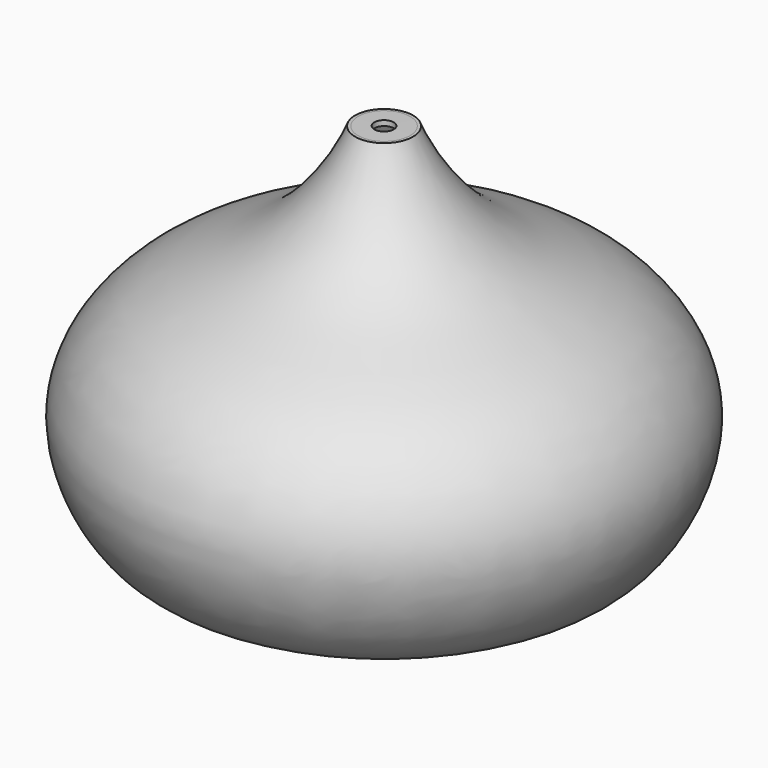
from build123d import *

# Parameters (mm, degrees)
F2_R     = 5
F3_DEPTH = 190


# Not quite as in the source:
# - ends of sketch curves that miss each other by under 0.0002 mm in the source are joined
# - the dataset's text gives a spline's control points without its knots; the knots are read off the source's solid


with BuildPart() as f1:
    # F0 (on Front) → F1 (revolve)
    with BuildSketch(Plane.XZ):
        with BuildLine():
            add(Edge.make_bspline(
                [(14.343489442, 187.2585117817), (14.2663053439, 187.4397829938), (14.1386699731, 187.7433208578), (13.9782055627, 188.1338468778), (13.8503601173, 188.4522717968), (13.7404223582, 188.7337167397), (13.6480782433, 188.9785031818), (13.5727745992, 189.1878497286), (13.5218227918, 189.3405777709), (13.486624217, 189.4573270267), (13.4553131706, 189.5742320778), (13.4263798732, 189.7229286458), (13.4157782973, 189.8307461373), (13.4130686106, 189.8717478482)],
                knots=[0.9558488315, 0.9558488315, 0.9558488315, 0.9558488315, 0.9609375, 0.96484375, 0.96875, 0.97265625, 0.9765625, 0.98046875, 0.984375, 0.986328125, 0.98828125, 0.990234375, 0.991435478, 0.991435478, 0.991435478, 0.991435478], degree=3))
            Line((13.4130686106, 189.8717478482), (0, 190))
            Line((0, 190), (0, 187.2585119684))
            Line((0, 187.2585119684), (14.343489442, 187.2585117817))
        make_face()
        with BuildLine():
            Line((95, 1.5), (95, 0))
            add(Edge.make_bspline(
                [(95, 0), (102.9937684759, 0), (122.9782858305, 10.509018894), (146.1044192238, 63.7249983964), (110.903188037, 115.1566102385), (51.7386639276, 132.8768445949), (21.5867324694, 173.4794491758), (15.1702392688, 189.0416115021), (14.9329743018, 189.857214919)],
                knots=[0, 0, 0, 0, 0.1330681946, 0.3176604379, 0.5074320376, 0.7085947345, 0.890855414, 0.9858462379, 0.9858462379, 0.9858462379, 0.9858462379], degree=3))
            Line((14.9329743018, 189.857214919), (13.4130686106, 189.8717478482))
            add(Edge.make_bspline(
                [(14.343489442, 187.2585117817), (14.2663053439, 187.4397829938), (14.1386699731, 187.7433208578), (13.9782055627, 188.1338468778), (13.8503601173, 188.4522717968), (13.7404223582, 188.7337167397), (13.6480782433, 188.9785031818), (13.5727745992, 189.1878497286), (13.5218227918, 189.3405777709), (13.486624217, 189.4573270267), (13.4553131706, 189.5742320778), (13.4263798732, 189.7229286458), (13.4157782973, 189.8307461373), (13.4130686106, 189.8717478482)],
                knots=[0.9558488315, 0.9558488315, 0.9558488315, 0.9558488315, 0.9609375, 0.96484375, 0.96875, 0.97265625, 0.9765625, 0.98046875, 0.984375, 0.986328125, 0.98828125, 0.990234375, 0.991435478, 0.991435478, 0.991435478, 0.991435478], degree=3))
            add(Edge.make_bspline(
                [(95, 1.5), (96.7479430492, 1.5), (100.2949587316, 1.9513666821), (105.7027636538, 3.985109507), (110.1992630606, 6.8153047921), (113.7325944043, 9.756852486), (116.3354116002, 12.2986877618), (118.8777838254, 15.176286785), (122.1591309147, 19.4399280718), (125.9739770946, 25.4758105315), (129.8530929693, 33.5750797312), (132.8005688925, 42.2533063451), (134.2923182137, 49.7368174104), (134.7976929983, 55.7363427659), (134.8077110706, 60.2086058663), (134.4181314867, 64.6189038237), (133.3724015126, 70.4183161076), (131.135276859, 77.4821784136), (127.1175641166, 85.5623366075), (121.9288336105, 93.1373866772), (116.7673996067, 98.9374575455), (112.2208964662, 103.2145172586), (108.6236738978, 106.2285110467), (104.8616019453, 109.0298270168), (99.639886693, 112.5068396641), (92.7871573199, 116.4560655612), (84.230308329, 120.8118284241), (75.532439228, 125.0437356242), (68.3276201418, 128.6870421823), (62.6868600605, 131.8062774523), (58.5426038885, 134.2826081268), (54.5087578983, 136.9284057607), (50.61368212, 139.7847382003), (46.8867439194, 142.8284621522), (42.1403589284, 147.0917773063), (36.6382830935, 152.7296280562), (30.7573371698, 159.7430580915), (26.4866934663, 165.5910946534), (23.4657622797, 170.1504762164), (21.4024609611, 173.4801240847), (19.5453483028, 176.6909739923), (17.9012318978, 179.7494525127), (16.7244789843, 182.0890600998), (15.9069715459, 183.7889080719), (15.3579150044, 184.9660869804), (14.8749513381, 186.0339908377), (14.5501338582, 186.7755651345), (14.3848040767, 187.1614820298), (14.343489442, 187.2585117817)],
                knots=[0, 0, 0, 0, 0.03125, 0.0625, 0.09375, 0.109375, 0.125, 0.140625, 0.15625, 0.1875, 0.21875, 0.25, 0.28125, 0.296875, 0.3125, 0.328125, 0.34375, 0.375, 0.40625, 0.4375, 0.46875, 0.484375, 0.5, 0.515625, 0.53125, 0.5625, 0.59375, 0.625, 0.65625, 0.671875, 0.6875, 0.703125, 0.71875, 0.734375, 0.75, 0.78125, 0.8125, 0.84375, 0.859375, 0.875, 0.890625, 0.90625, 0.921875, 0.9296875, 0.9375, 0.9453125, 0.953125, 0.9558488315, 0.9558488315, 0.9558488315, 0.9558488315], degree=3))
        make_face()
    revolve(axis=Axis((0, 0, 95), (0, 0, 1)))

    # F2 (on Top) → F3 (cut)
    with BuildSketch(Plane.XY):
        Circle(F2_R)
    extrude(amount=F3_DEPTH, mode=Mode.SUBTRACT)


solid = f1.part
